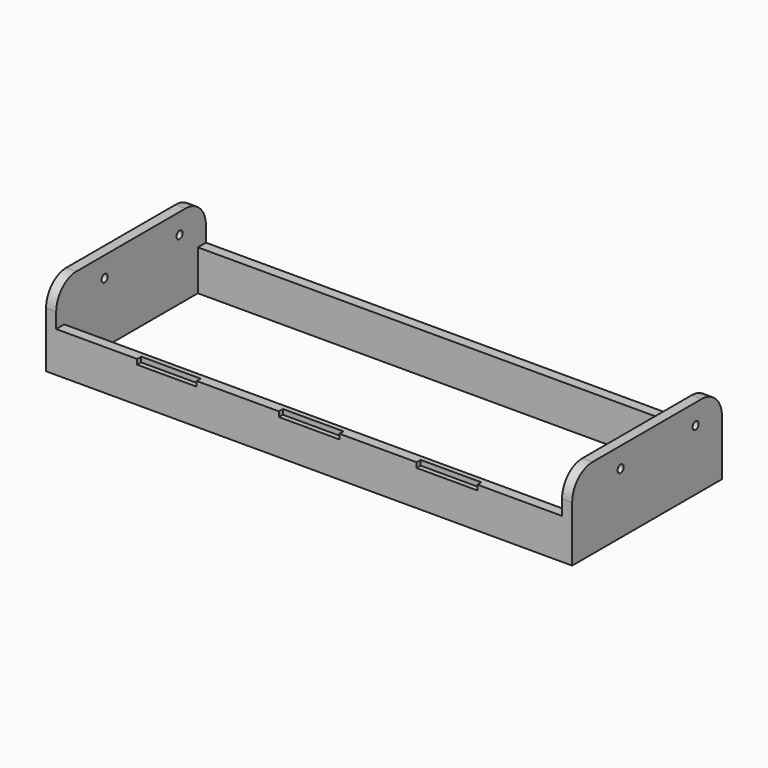
from build123d import *

# Parameters (mm, degrees)
F0_W          = 104
F0_H          = 37
F0_W_2        = 100
F0_H_2        = 33
F1_DEPTH      = 8
F3_DEPTH      = 1
F5_DEPTH      = 8
F6_R          = 0.75
F7_DEPTH      = 10.7
F7_DEPTH_BACK = 110.5
F8_R          = 5


with BuildPart() as f1:
    # F0 (on Top) → F1 (new body)
    with BuildSketch(Plane.XY):
        with Locations((52, 18.5)):
            Rectangle(F0_W, F0_H)
        with Locations((52, 18.5)):
            Rectangle(F0_W_2, F0_H_2, mode=Mode.SUBTRACT)
    extrude(amount=F1_DEPTH)

    # F2 (on face) → F3 (cut)
    with BuildSketch(Plane.XY.offset(8)):
        Polygon((46, 0), (52, 0), (58, 0), (58, 1), (52, 1), (46, 1), align=None)
        Polygon((18, 0), (24, 0), (29.75, 0), (29.75, 1), (23.75, 1), (18, 1), align=None)
        Polygon((73.25, 0), (80, 0), (85.25, 0), (85.25, 1), (79.25, 1), (73.25, 1), align=None)
    extrude(amount=-F3_DEPTH, mode=Mode.SUBTRACT)

    # F4 (on face) → F5 (join)
    with BuildSketch(Plane.XY.offset(8)):
        Polygon((0, 37), (0, 0), (2, 0), (2, 2), (2, 35), (2, 37), align=None)
        Polygon((104, 37), (102, 37), (102, 35), (102, 2), (102, 0), (104, 0), align=None)
    extrude(amount=F5_DEPTH)

    # F6 (on face) → F7 (cut, two sides)
    with BuildSketch(Plane(origin=(102, 0, 0), x_dir=(0, -1, 0), z_dir=(-1, 0, 0))) as f7_sk:
        with Locations((-30.5038709193, 12)):
            Circle(F6_R)
        with Locations((-11.9723072276, 12)):
            Circle(F6_R)
    extrude(amount=-F7_DEPTH, mode=Mode.SUBTRACT)
    extrude(f7_sk.sketch, amount=F7_DEPTH_BACK, mode=Mode.SUBTRACT)

    # F8
    f8_edges = [f1.edges().sort_by_distance(p)[0] for p in [
        (1, 0, 16),
        (103, 0, 16),
        (103, 37, 16),
        (1, 37, 16),
    ]]
    fillet(f8_edges, radius=F8_R)


solid = f1.part
